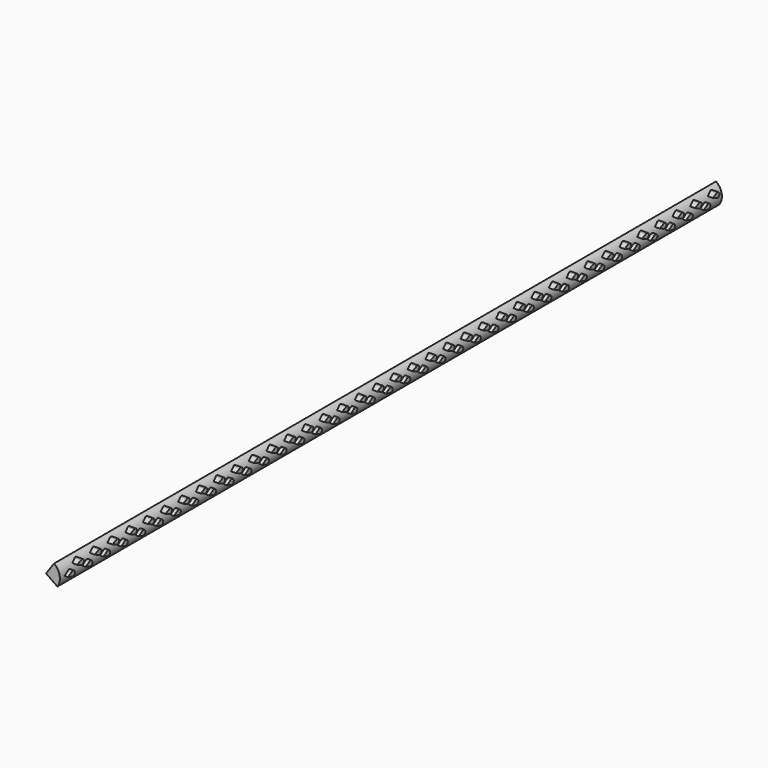
from build123d import *

# Parameters (mm, degrees)
F1_DEPTH = 3000
F4_DEPTH = 12.5


# Not quite as in the source:
# - a feature names something its author has since deleted; it is built from what else it names


with BuildPart() as f1:
    # F0 (on Front) → F1 (new body)
    with BuildSketch(Plane.XZ):
        with BuildLine():
            Line((0, 0), (40.9576022144, -28.6788218176))
            ThreePointArc((40.9576022144, -28.6788218176), (49.2403876506, 8.6824088833), (28.6788218176, 40.9576022144))
            Line((28.6788218176, 40.9576022144), (0, 0))
        make_face()
    extrude(amount=-F1_DEPTH)

    # F3 (on offset) → F4 (join, symmetric)
    with BuildSketch(Plane.YZ.offset(50)):
        with BuildLine():
            Line((38.7130560613, 10.2562727251), (21.543056941, 0))
            Line((21.543056941, 0), (40.620881733, -6.0030493256))
            ThreePointArc((40.620881733, -6.0030493256), (52.3216302546, 3.6114760581), (38.7130560613, 10.2562727251))
        make_face()
        with BuildLine():
            Line((198.7130560613, 10.2562727251), (181.543056941, 0))
            Line((181.543056941, 0), (200.620881733, -6.0030493256))
            ThreePointArc((200.620881733, -6.0030493256), (212.3216302546, 3.6114760581), (198.7130560613, 10.2562727251))
        make_face()
        with BuildLine():
            Line((278.7130560613, 10.2562727251), (261.543056941, 0))
            Line((261.543056941, 0), (280.620881733, -6.0030493256))
            ThreePointArc((280.620881733, -6.0030493256), (292.3216302546, 3.6114760581), (278.7130560613, 10.2562727251))
        make_face()
        with BuildLine():
            Line((358.7130560613, 10.2562727251), (341.543056941, 0))
            Line((341.543056941, 0), (360.620881733, -6.0030493256))
            ThreePointArc((360.620881733, -6.0030493256), (372.3216302546, 3.6114760581), (358.7130560613, 10.2562727251))
        make_face()
        with BuildLine():
            Line((438.7130560613, 10.2562727251), (421.543056941, 0))
            Line((421.543056941, 0), (440.620881733, -6.0030493256))
            ThreePointArc((440.620881733, -6.0030493256), (452.3216302546, 3.6114760581), (438.7130560613, 10.2562727251))
        make_face()
        with BuildLine():
            Line((518.7130560613, 10.2562727251), (501.543056941, 0))
            Line((501.543056941, 0), (520.620881733, -6.0030493256))
            ThreePointArc((520.620881733, -6.0030493256), (532.3216302546, 3.6114760581), (518.7130560613, 10.2562727251))
        make_face()
        with BuildLine():
            Line((598.7130560613, 10.2562727251), (581.543056941, 0))
            Line((581.543056941, 0), (600.620881733, -6.0030493256))
            ThreePointArc((600.620881733, -6.0030493256), (612.3216302546, 3.6114760581), (598.7130560613, 10.2562727251))
        make_face()
        with BuildLine():
            Line((678.7130560613, 10.2562727251), (661.543056941, 0))
            Line((661.543056941, 0), (680.620881733, -6.0030493256))
            ThreePointArc((680.620881733, -6.0030493256), (692.3216302546, 3.6114760581), (678.7130560613, 10.2562727251))
        make_face()
        with BuildLine():
            Line((758.7130560613, 10.2562727251), (741.543056941, 0))
            Line((741.543056941, 0), (760.620881733, -6.0030493256))
            ThreePointArc((760.620881733, -6.0030493256), (772.3216302546, 3.6114760581), (758.7130560613, 10.2562727251))
        make_face()
        with BuildLine():
            Line((838.7130560613, 10.2562727251), (821.543056941, 0))
            Line((821.543056941, 0), (840.620881733, -6.0030493256))
            ThreePointArc((840.620881733, -6.0030493256), (852.3216302546, 3.6114760581), (838.7130560613, 10.2562727251))
        make_face()
        with BuildLine():
            Line((118.7130560613, 10.2562727251), (101.543056941, 0))
            Line((101.543056941, 0), (120.620881733, -6.0030493256))
            ThreePointArc((120.620881733, -6.0030493256), (132.3216302546, 3.6114760581), (118.7130560613, 10.2562727251))
        make_face()
        with BuildLine():
            Line((918.7130560613, 10.2562727251), (901.543056941, 0))
            Line((901.543056941, 0), (920.620881733, -6.0030493256))
            ThreePointArc((920.620881733, -6.0030493256), (932.3216302546, 3.6114760581), (918.7130560613, 10.2562727251))
        make_face()
        with BuildLine():
            Line((998.7130560613, 10.2562727251), (981.543056941, 0))
            Line((981.543056941, 0), (1000.620881733, -6.0030493256))
            ThreePointArc((1000.620881733, -6.0030493256), (1012.3216302546, 3.6114760581), (998.7130560613, 10.2562727251))
        make_face()
        with BuildLine():
            Line((1078.7130560613, 10.2562727251), (1061.543056941, 0))
            Line((1061.543056941, 0), (1080.620881733, -6.0030493256))
            ThreePointArc((1080.620881733, -6.0030493256), (1092.3216302546, 3.6114760581), (1078.7130560613, 10.2562727251))
        make_face()
        with BuildLine():
            Line((1158.7130560613, 10.2562727251), (1141.543056941, 0))
            Line((1141.543056941, 0), (1160.620881733, -6.0030493256))
            ThreePointArc((1160.620881733, -6.0030493256), (1172.3216302546, 3.6114760581), (1158.7130560613, 10.2562727251))
        make_face()
        with BuildLine():
            Line((1318.7130560613, 10.2562727251), (1301.543056941, 0))
            Line((1301.543056941, 0), (1320.620881733, -6.0030493256))
            ThreePointArc((1320.620881733, -6.0030493256), (1332.3216302546, 3.6114760581), (1318.7130560613, 10.2562727251))
        make_face()
        with BuildLine():
            Line((1398.7130560613, 10.2562727251), (1381.543056941, 0))
            Line((1381.543056941, 0), (1400.620881733, -6.0030493256))
            ThreePointArc((1400.620881733, -6.0030493256), (1412.3216302546, 3.6114760581), (1398.7130560613, 10.2562727251))
        make_face()
        with BuildLine():
            Line((1478.7130560613, 10.2562727251), (1461.543056941, 0))
            Line((1461.543056941, 0), (1480.620881733, -6.0030493256))
            ThreePointArc((1480.620881733, -6.0030493256), (1492.3216302546, 3.6114760581), (1478.7130560613, 10.2562727251))
        make_face()
        with BuildLine():
            Line((1558.7130560613, 10.2562727251), (1541.543056941, 0))
            Line((1541.543056941, 0), (1560.620881733, -6.0030493256))
            ThreePointArc((1560.620881733, -6.0030493256), (1572.3216302546, 3.6114760581), (1558.7130560613, 10.2562727251))
        make_face()
        with BuildLine():
            Line((1638.7130560613, 10.2562727251), (1621.543056941, 0))
            Line((1621.543056941, 0), (1640.620881733, -6.0030493256))
            ThreePointArc((1640.620881733, -6.0030493256), (1652.3216302546, 3.6114760581), (1638.7130560613, 10.2562727251))
        make_face()
        with BuildLine():
            Line((1718.7130560613, 10.2562727251), (1701.543056941, 0))
            Line((1701.543056941, 0), (1720.620881733, -6.0030493256))
            ThreePointArc((1720.620881733, -6.0030493256), (1732.3216302546, 3.6114760581), (1718.7130560613, 10.2562727251))
        make_face()
        with BuildLine():
            Line((1798.7130560613, 10.2562727251), (1781.543056941, 0))
            Line((1781.543056941, 0), (1800.620881733, -6.0030493256))
            ThreePointArc((1800.620881733, -6.0030493256), (1812.3216302546, 3.6114760581), (1798.7130560613, 10.2562727251))
        make_face()
        with BuildLine():
            Line((1878.7130560613, 10.2562727251), (1861.543056941, 0))
            Line((1861.543056941, 0), (1880.620881733, -6.0030493256))
            ThreePointArc((1880.620881733, -6.0030493256), (1892.3216302546, 3.6114760581), (1878.7130560613, 10.2562727251))
        make_face()
        with BuildLine():
            Line((1958.7130560613, 10.2562727251), (1941.543056941, 0))
            Line((1941.543056941, 0), (1960.620881733, -6.0030493256))
            ThreePointArc((1960.620881733, -6.0030493256), (1972.3216302546, 3.6114760581), (1958.7130560613, 10.2562727251))
        make_face()
        with BuildLine():
            Line((2038.7130560613, 10.2562727251), (2021.543056941, 0))
            Line((2021.543056941, 0), (2040.620881733, -6.0030493256))
            ThreePointArc((2040.620881733, -6.0030493256), (2052.3216302546, 3.6114760581), (2038.7130560613, 10.2562727251))
        make_face()
        with BuildLine():
            Line((2118.7130560613, 10.2562727251), (2101.543056941, 0))
            Line((2101.543056941, 0), (2120.620881733, -6.0030493256))
            ThreePointArc((2120.620881733, -6.0030493256), (2132.3216302546, 3.6114760581), (2118.7130560613, 10.2562727251))
        make_face()
        with BuildLine():
            Line((2198.7130560613, 10.2562727251), (2181.543056941, 0))
            Line((2181.543056941, 0), (2200.620881733, -6.0030493256))
            ThreePointArc((2200.620881733, -6.0030493256), (2212.3216302546, 3.6114760581), (2198.7130560613, 10.2562727251))
        make_face()
        with BuildLine():
            Line((2278.7130560613, 10.2562727251), (2261.543056941, 0))
            Line((2261.543056941, 0), (2280.620881733, -6.0030493256))
            ThreePointArc((2280.620881733, -6.0030493256), (2292.3216302546, 3.6114760581), (2278.7130560613, 10.2562727251))
        make_face()
        with BuildLine():
            Line((1238.7130560613, 10.2562727251), (1221.543056941, 0))
            Line((1221.543056941, 0), (1240.620881733, -6.0030493256))
            ThreePointArc((1240.620881733, -6.0030493256), (1252.3216302546, 3.6114760581), (1238.7130560613, 10.2562727251))
        make_face()
        with BuildLine():
            Line((2358.7130560613, 10.2562727251), (2341.543056941, 0))
            Line((2341.543056941, 0), (2360.620881733, -6.0030493256))
            ThreePointArc((2360.620881733, -6.0030493256), (2372.3216302546, 3.6114760581), (2358.7130560613, 10.2562727251))
        make_face()
        with BuildLine():
            Line((2438.7130560613, 10.2562727251), (2421.543056941, 0))
            Line((2421.543056941, 0), (2440.620881733, -6.0030493256))
            ThreePointArc((2440.620881733, -6.0030493256), (2452.3216302546, 3.6114760581), (2438.7130560613, 10.2562727251))
        make_face()
        with BuildLine():
            Line((2518.7130560613, 10.2562727251), (2501.543056941, 0))
            Line((2501.543056941, 0), (2520.620881733, -6.0030493256))
            ThreePointArc((2520.620881733, -6.0030493256), (2532.3216302546, 3.6114760581), (2518.7130560613, 10.2562727251))
        make_face()
        with BuildLine():
            Line((2598.7130560613, 10.2562727251), (2581.543056941, 0))
            Line((2581.543056941, 0), (2600.620881733, -6.0030493256))
            ThreePointArc((2600.620881733, -6.0030493256), (2612.3216302546, 3.6114760581), (2598.7130560613, 10.2562727251))
        make_face()
        with BuildLine():
            Line((2678.7130560613, 10.2562727251), (2661.543056941, 0))
            Line((2661.543056941, 0), (2680.620881733, -6.0030493256))
            ThreePointArc((2680.620881733, -6.0030493256), (2692.3216302546, 3.6114760581), (2678.7130560613, 10.2562727251))
        make_face()
        with BuildLine():
            Line((2758.7130560613, 10.2562727251), (2741.543056941, 0))
            Line((2741.543056941, 0), (2760.620881733, -6.0030493256))
            ThreePointArc((2760.620881733, -6.0030493256), (2772.3216302546, 3.6114760581), (2758.7130560613, 10.2562727251))
        make_face()
        with BuildLine():
            Line((2838.7130560613, 10.2562727251), (2821.543056941, 0))
            Line((2821.543056941, 0), (2840.620881733, -6.0030493256))
            ThreePointArc((2840.620881733, -6.0030493256), (2852.3216302546, 3.6114760581), (2838.7130560613, 10.2562727251))
        make_face()
        with BuildLine():
            Line((2918.7130560613, 10.2562727251), (2901.543056941, 0))
            Line((2901.543056941, 0), (2920.620881733, -6.0030493256))
            ThreePointArc((2920.620881733, -6.0030493256), (2932.3216302546, 3.6114760581), (2918.7130560613, 10.2562727251))
        make_face()
        with BuildLine():
            Line((80.6213840842, 30.5932002939), (62.3829539807, 22.3859067474))
            Line((62.3829539807, 22.3859067474), (80.6213840842, 14.1786132008))
            ThreePointArc((80.6213840842, 14.1786132008), (93.3146661802, 22.3859067474), (80.6213840842, 30.5932002939))
        make_face()
        with BuildLine():
            Line((160.6213840842, 30.5932002939), (142.3829539807, 22.3859067474))
            Line((142.3829539807, 22.3859067474), (160.6213840842, 14.1786132008))
            ThreePointArc((160.6213840842, 14.1786132008), (173.3146661802, 22.3859067474), (160.6213840842, 30.5932002939))
        make_face()
        with BuildLine():
            Line((240.6213840842, 30.5932002939), (222.3829539807, 22.3859067474))
            Line((222.3829539807, 22.3859067474), (240.6213840842, 14.1786132008))
            ThreePointArc((240.6213840842, 14.1786132008), (253.3146661802, 22.3859067474), (240.6213840842, 30.5932002939))
        make_face()
        with BuildLine():
            Line((320.6213840842, 30.5932002939), (302.3829539807, 22.3859067474))
            Line((302.3829539807, 22.3859067474), (320.6213840842, 14.1786132008))
            ThreePointArc((320.6213840842, 14.1786132008), (333.3146661802, 22.3859067474), (320.6213840842, 30.5932002939))
        make_face()
        with BuildLine():
            Line((400.6213840842, 30.5932002939), (382.3829539807, 22.3859067474))
            Line((382.3829539807, 22.3859067474), (400.6213840842, 14.1786132008))
            ThreePointArc((400.6213840842, 14.1786132008), (413.3146661802, 22.3859067474), (400.6213840842, 30.5932002939))
        make_face()
        with BuildLine():
            Line((480.6213840842, 30.5932002939), (462.3829539807, 22.3859067474))
            Line((462.3829539807, 22.3859067474), (480.6213840842, 14.1786132008))
            ThreePointArc((480.6213840842, 14.1786132008), (493.3146661802, 22.3859067474), (480.6213840842, 30.5932002939))
        make_face()
        with BuildLine():
            Line((560.6213840842, 30.5932002939), (542.3829539807, 22.3859067474))
            Line((542.3829539807, 22.3859067474), (560.6213840842, 14.1786132008))
            ThreePointArc((560.6213840842, 14.1786132008), (573.3146661802, 22.3859067474), (560.6213840842, 30.5932002939))
        make_face()
        with BuildLine():
            Line((640.6213840842, 30.5932002939), (622.3829539807, 22.3859067474))
            Line((622.3829539807, 22.3859067474), (640.6213840842, 14.1786132008))
            ThreePointArc((640.6213840842, 14.1786132008), (653.3146661802, 22.3859067474), (640.6213840842, 30.5932002939))
        make_face()
        with BuildLine():
            Line((720.6213840842, 30.5932002939), (702.3829539807, 22.3859067474))
            Line((702.3829539807, 22.3859067474), (720.6213840842, 14.1786132008))
            ThreePointArc((720.6213840842, 14.1786132008), (733.3146661802, 22.3859067474), (720.6213840842, 30.5932002939))
        make_face()
        with BuildLine():
            Line((800.6213840842, 30.5932002939), (782.3829539807, 22.3859067474))
            Line((782.3829539807, 22.3859067474), (800.6213840842, 14.1786132008))
            ThreePointArc((800.6213840842, 14.1786132008), (813.3146661802, 22.3859067474), (800.6213840842, 30.5932002939))
        make_face()
        with BuildLine():
            Line((880.6213840842, 30.5932002939), (862.3829539807, 22.3859067474))
            Line((862.3829539807, 22.3859067474), (880.6213840842, 14.1786132008))
            ThreePointArc((880.6213840842, 14.1786132008), (893.3146661802, 22.3859067474), (880.6213840842, 30.5932002939))
        make_face()
        with BuildLine():
            Line((960.6213840842, 30.5932002939), (942.3829539807, 22.3859067474))
            Line((942.3829539807, 22.3859067474), (960.6213840842, 14.1786132008))
            ThreePointArc((960.6213840842, 14.1786132008), (973.3146661802, 22.3859067474), (960.6213840842, 30.5932002939))
        make_face()
        with BuildLine():
            Line((1040.6213840842, 30.5932002939), (1022.3829539807, 22.3859067474))
            Line((1022.3829539807, 22.3859067474), (1040.6213840842, 14.1786132008))
            ThreePointArc((1040.6213840842, 14.1786132008), (1053.3146661802, 22.3859067474), (1040.6213840842, 30.5932002939))
        make_face()
        with BuildLine():
            Line((1120.6213840842, 30.5932002939), (1102.3829539807, 22.3859067474))
            Line((1102.3829539807, 22.3859067474), (1120.6213840842, 14.1786132008))
            ThreePointArc((1120.6213840842, 14.1786132008), (1133.3146661802, 22.3859067474), (1120.6213840842, 30.5932002939))
        make_face()
        with BuildLine():
            Line((1200.6213840842, 30.5932002939), (1182.3829539807, 22.3859067474))
            Line((1182.3829539807, 22.3859067474), (1200.6213840842, 14.1786132008))
            ThreePointArc((1200.6213840842, 14.1786132008), (1213.3146661802, 22.3859067474), (1200.6213840842, 30.5932002939))
        make_face()
        with BuildLine():
            Line((1280.6213840842, 30.5932002939), (1262.3829539807, 22.3859067474))
            Line((1262.3829539807, 22.3859067474), (1280.6213840842, 14.1786132008))
            ThreePointArc((1280.6213840842, 14.1786132008), (1293.3146661802, 22.3859067474), (1280.6213840842, 30.5932002939))
        make_face()
        with BuildLine():
            Line((1360.6213840842, 30.5932002939), (1342.3829539807, 22.3859067474))
            Line((1342.3829539807, 22.3859067474), (1360.6213840842, 14.1786132008))
            ThreePointArc((1360.6213840842, 14.1786132008), (1373.3146661802, 22.3859067474), (1360.6213840842, 30.5932002939))
        make_face()
        with BuildLine():
            Line((1440.6213840842, 30.5932002939), (1422.3829539807, 22.3859067474))
            Line((1422.3829539807, 22.3859067474), (1440.6213840842, 14.1786132008))
            ThreePointArc((1440.6213840842, 14.1786132008), (1453.3146661802, 22.3859067474), (1440.6213840842, 30.5932002939))
        make_face()
        with BuildLine():
            Line((1520.6213840842, 30.5932002939), (1502.3829539807, 22.3859067474))
            Line((1502.3829539807, 22.3859067474), (1520.6213840842, 14.1786132008))
            ThreePointArc((1520.6213840842, 14.1786132008), (1533.3146661802, 22.3859067474), (1520.6213840842, 30.5932002939))
        make_face()
        with BuildLine():
            Line((1600.6213840842, 30.5932002939), (1582.3829539807, 22.3859067474))
            Line((1582.3829539807, 22.3859067474), (1600.6213840842, 14.1786132008))
            ThreePointArc((1600.6213840842, 14.1786132008), (1613.3146661802, 22.3859067474), (1600.6213840842, 30.5932002939))
        make_face()
        with BuildLine():
            Line((1680.6213840842, 30.5932002939), (1662.3829539807, 22.3859067474))
            Line((1662.3829539807, 22.3859067474), (1680.6213840842, 14.1786132008))
            ThreePointArc((1680.6213840842, 14.1786132008), (1693.3146661802, 22.3859067474), (1680.6213840842, 30.5932002939))
        make_face()
        with BuildLine():
            Line((1760.6213840842, 30.5932002939), (1742.3829539807, 22.3859067474))
            Line((1742.3829539807, 22.3859067474), (1760.6213840842, 14.1786132008))
            ThreePointArc((1760.6213840842, 14.1786132008), (1773.3146661802, 22.3859067474), (1760.6213840842, 30.5932002939))
        make_face()
        with BuildLine():
            Line((1840.6213840842, 30.5932002939), (1822.3829539807, 22.3859067474))
            Line((1822.3829539807, 22.3859067474), (1840.6213840842, 14.1786132008))
            ThreePointArc((1840.6213840842, 14.1786132008), (1853.3146661802, 22.3859067474), (1840.6213840842, 30.5932002939))
        make_face()
        with BuildLine():
            Line((1920.6213840842, 30.5932002939), (1902.3829539807, 22.3859067474))
            Line((1902.3829539807, 22.3859067474), (1920.6213840842, 14.1786132008))
            ThreePointArc((1920.6213840842, 14.1786132008), (1933.3146661802, 22.3859067474), (1920.6213840842, 30.5932002939))
        make_face()
        with BuildLine():
            Line((2000.6213840842, 30.5932002939), (1982.3829539807, 22.3859067474))
            Line((1982.3829539807, 22.3859067474), (2000.6213840842, 14.1786132008))
            ThreePointArc((2000.6213840842, 14.1786132008), (2013.3146661802, 22.3859067474), (2000.6213840842, 30.5932002939))
        make_face()
        with BuildLine():
            Line((2160.6213840842, 30.5932002939), (2142.3829539807, 22.3859067474))
            Line((2142.3829539807, 22.3859067474), (2160.6213840842, 14.1786132008))
            ThreePointArc((2160.6213840842, 14.1786132008), (2173.3146661802, 22.3859067474), (2160.6213840842, 30.5932002939))
        make_face()
        with BuildLine():
            Line((2240.6213840842, 30.5932002939), (2222.3829539807, 22.3859067474))
            Line((2222.3829539807, 22.3859067474), (2240.6213840842, 14.1786132008))
            ThreePointArc((2240.6213840842, 14.1786132008), (2253.3146661802, 22.3859067474), (2240.6213840842, 30.5932002939))
        make_face()
        with BuildLine():
            Line((2320.6213840842, 30.5932002939), (2302.3829539807, 22.3859067474))
            Line((2302.3829539807, 22.3859067474), (2320.6213840842, 14.1786132008))
            ThreePointArc((2320.6213840842, 14.1786132008), (2333.3146661802, 22.3859067474), (2320.6213840842, 30.5932002939))
        make_face()
        with BuildLine():
            Line((2400.6213840842, 30.5932002939), (2382.3829539807, 22.3859067474))
            Line((2382.3829539807, 22.3859067474), (2400.6213840842, 14.1786132008))
            ThreePointArc((2400.6213840842, 14.1786132008), (2413.3146661802, 22.3859067474), (2400.6213840842, 30.5932002939))
        make_face()
        with BuildLine():
            Line((2640.6213840842, 30.5932002939), (2622.3829539807, 22.3859067474))
            Line((2622.3829539807, 22.3859067474), (2640.6213840842, 14.1786132008))
            ThreePointArc((2640.6213840842, 14.1786132008), (2653.3146661802, 22.3859067474), (2640.6213840842, 30.5932002939))
        make_face()
        with BuildLine():
            Line((2720.6213840842, 30.5932002939), (2702.3829539807, 22.3859067474))
            Line((2702.3829539807, 22.3859067474), (2720.6213840842, 14.1786132008))
            ThreePointArc((2720.6213840842, 14.1786132008), (2733.3146661802, 22.3859067474), (2720.6213840842, 30.5932002939))
        make_face()
        with BuildLine():
            Line((2800.6213840842, 30.5932002939), (2782.3829539807, 22.3859067474))
            Line((2782.3829539807, 22.3859067474), (2800.6213840842, 14.1786132008))
            ThreePointArc((2800.6213840842, 14.1786132008), (2813.3146661802, 22.3859067474), (2800.6213840842, 30.5932002939))
        make_face()
        with BuildLine():
            Line((2880.6213840842, 30.5932002939), (2862.3829539807, 22.3859067474))
            Line((2862.3829539807, 22.3859067474), (2880.6213840842, 14.1786132008))
            ThreePointArc((2880.6213840842, 14.1786132008), (2893.3146661802, 22.3859067474), (2880.6213840842, 30.5932002939))
        make_face()
        with BuildLine():
            Line((2960.6213840842, 30.5932002939), (2942.3829539807, 22.3859067474))
            Line((2942.3829539807, 22.3859067474), (2960.6213840842, 14.1786132008))
            ThreePointArc((2960.6213840842, 14.1786132008), (2973.3146661802, 22.3859067474), (2960.6213840842, 30.5932002939))
        make_face()
        with BuildLine():
            Line((2080.6213840842, 30.5932002939), (2062.3829539807, 22.3859067474))
            Line((2062.3829539807, 22.3859067474), (2080.6213840842, 14.1786132008))
            ThreePointArc((2080.6213840842, 14.1786132008), (2093.3146661802, 22.3859067474), (2080.6213840842, 30.5932002939))
        make_face()
        with BuildLine():
            Line((2480.6213840842, 30.5932002939), (2462.3829539807, 22.3859067474))
            Line((2462.3829539807, 22.3859067474), (2480.6213840842, 14.1786132008))
            ThreePointArc((2480.6213840842, 14.1786132008), (2493.3146661802, 22.3859067474), (2480.6213840842, 30.5932002939))
        make_face()
        with BuildLine():
            Line((2560.6213840842, 30.5932002939), (2542.3829539807, 22.3859067474))
            Line((2542.3829539807, 22.3859067474), (2560.6213840842, 14.1786132008))
            ThreePointArc((2560.6213840842, 14.1786132008), (2573.3146661802, 22.3859067474), (2560.6213840842, 30.5932002939))
        make_face()
    extrude(amount=F4_DEPTH, both=True)


solid = f1.part
